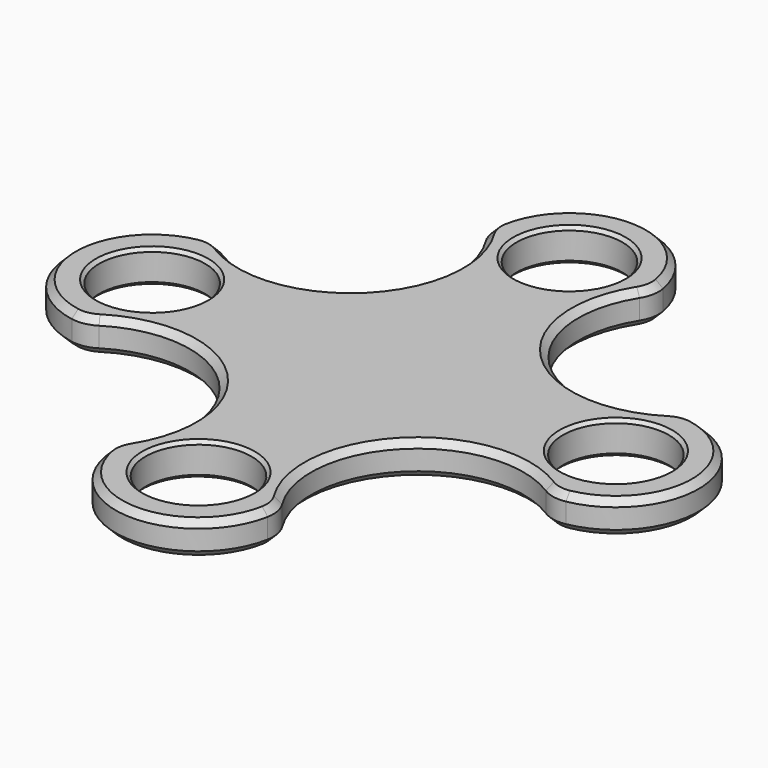
from build123d import *

# Parameters (mm, degrees)
F0_R     = 8
F1_DEPTH = 5
F2_SIZE  = 1
F3_SIZE  = 0.5


# Not quite as in the source:
# - a feature names something its author has since deleted; it is built from what else it names


with BuildPart() as f1:
    # F0 (on Top) → F1 (new body)
    with BuildSketch(Plane.XY):
        with BuildLine():
            ThreePointArc((11.6083434008, 33.7208583728), (12.2845984061, 35.4442804748), (12.2873952004, 37.2956304556))
            ThreePointArc((12.2873952004, 37.2956304556), (0, 47.5), (-12.2873952004, 37.2956304556))
            ThreePointArc((-12.2873952004, 37.2956304556), (-12.2845984061, 35.4442804748), (-11.6083434008, 33.7208583728))
            ThreePointArc((-11.6083434008, 33.7208583728), (-13.8553017596, 13.8553017596), (-33.7208583728, 11.6083434008))
            ThreePointArc((-33.7208583728, 11.6083434008), (-35.4442804748, 12.2845984061), (-37.2956304556, 12.2873952004))
            ThreePointArc((-37.2956304556, 12.2873952004), (-47.5, 0), (-37.2956304556, -12.2873952004))
            ThreePointArc((-37.2956304556, -12.2873952004), (-35.4442804748, -12.2845984061), (-33.7208583728, -11.6083434008))
            ThreePointArc((-33.7208583728, -11.6083434008), (-13.8553017596, -13.8553017596), (-11.6083434008, -33.7208583728))
            ThreePointArc((-11.6083434008, -33.7208583728), (-12.2845984061, -35.4442804748), (-12.2873952004, -37.2956304556))
            ThreePointArc((-12.2873952004, -37.2956304556), (0, -47.5), (12.2873952004, -37.2956304556))
            ThreePointArc((12.2873952004, -37.2956304556), (12.2845984061, -35.4442804748), (11.6083434008, -33.7208583728))
            ThreePointArc((11.6083434008, -33.7208583728), (13.8553017596, -13.8553017596), (33.7208583728, -11.6083434008))
            ThreePointArc((33.7208583728, -11.6083434008), (35.4442804748, -12.2845984061), (37.2956304556, -12.2873952004))
            ThreePointArc((37.2956304556, -12.2873952004), (47.5, 0), (37.2956304556, 12.2873952004))
            ThreePointArc((37.2956304556, 12.2873952004), (35.4442804748, 12.2845984061), (33.7208583728, 11.6083434008))
            ThreePointArc((33.7208583728, 11.6083434008), (13.8553017596, 13.8553017596), (11.6083434008, 33.7208583728))
        make_face()
        with Locations((0, -35)):
            Circle(F0_R, mode=Mode.SUBTRACT)
        with Locations((-35, 0)):
            Circle(F0_R, mode=Mode.SUBTRACT)
        with Locations((35, 0)):
            Circle(F0_R, mode=Mode.SUBTRACT)
        with Locations((0, 35)):
            Circle(F0_R, mode=Mode.SUBTRACT)
    extrude(amount=F1_DEPTH)

    # F2
    f2_edges = [f1.edges().sort_by_distance(p)[0] for p in [
        (-47.5, 0, 5),
        (-13.855302, -13.855302, 5),
        (-13.855302, 13.855302, 5),
        (0, 47.5, 5),
        (13.855302, 13.855302, 5),
        (47.5, 0, 5),
        (13.855302, -13.855302, 5),
        (0, -47.5, 5),
        (13.855302, 13.855302, 0),
        (0, 47.5, 0),
        (-13.855302, 13.855302, 0),
        (-47.5, 0, 0),
        (-13.855302, -13.855302, 0),
        (0, -47.5, 0),
        (13.855302, -13.855302, 0),
        (47.5, 0, 0),
    ]]
    chamfer(f2_edges, length=F2_SIZE)

    # F3
    f3_edges = [f1.edges().sort_by_distance(p)[0] for p in [
        (-8, 35, 5),
        (-8, -35, 5),
        (27, 0, 5),
        (-43, 0, 5),
        (-8, 35, 0),
        (-43, 0, 0),
        (27, 0, 0),
        (-8, -35, 0),
    ]]
    chamfer(f3_edges, length=F3_SIZE)


solid = f1.part
